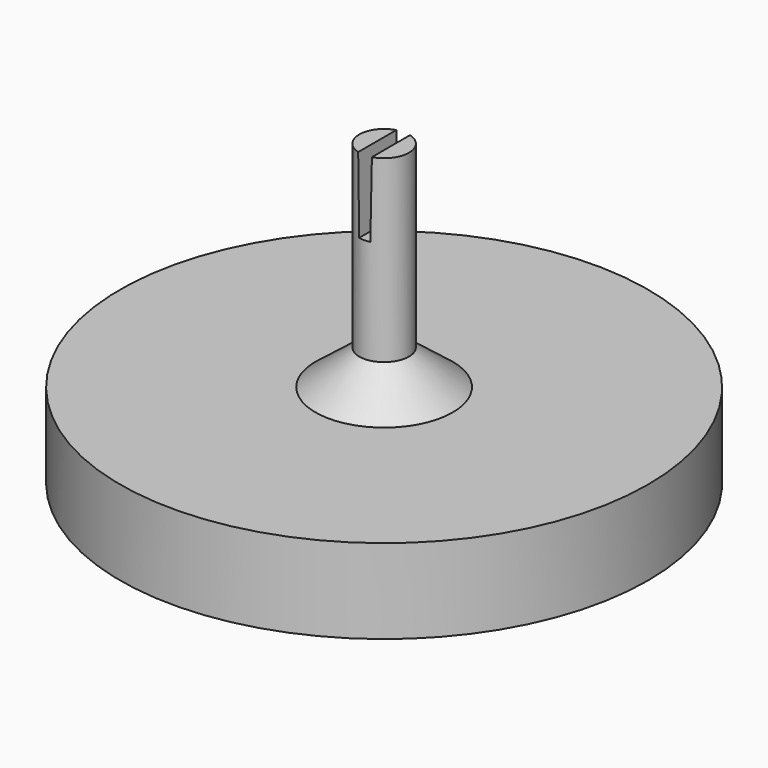
from build123d import *

# Parameters (mm, degrees)
F0_R      = 25
F1_DEPTH  = 8
F2_R      = 20.675
F3_DEPTH  = 4
F4_R      = 6.95
F5_DEPTH  = 1
F6_R      = 6.5
F7_DEPTH  = 3.3
F7_TAPER  = 52
F8_R      = 2.35
F9_DEPTH  = 17
F11_DEPTH = 7.1
F11_TAPER = 1


# Not quite as in the source:
# - a feature names something its author has since deleted; it is built from what else it names


with BuildPart() as f1:
    # F0 (on Top) → F1 (new body)
    with BuildSketch(Plane.XY):
        Circle(F0_R)
    extrude(amount=F1_DEPTH)

    # F2 (on face) → F3 (cut)
    with BuildSketch(Plane(origin=(0, 0, 0), x_dir=(1, 0, 0), z_dir=(0, 0, -1))):
        Circle(F2_R)
    extrude(amount=-F3_DEPTH, mode=Mode.SUBTRACT)

    # F4 (on face) → F5 (cut)
    with BuildSketch(Plane(origin=(0, 0, 4), x_dir=(1, 0, 0), z_dir=(0, 0, -1))):
        Circle(F4_R)
    extrude(amount=-F5_DEPTH, mode=Mode.SUBTRACT)

    # F6 (on face) → F7 (join)
    with BuildSketch(Plane.XY.offset(8)):
        Circle(F6_R)
    extrude(amount=F7_DEPTH, taper=F7_TAPER)

    # F8 (on face) → F9 (join)
    with BuildSketch(Plane.XY.offset(11.3)):
        Circle(F8_R)
    extrude(amount=F9_DEPTH)

    # F10 (on face) → F11 (cut)
    with BuildSketch(Plane.XY.offset(28.3)):
        with BuildLine():
            ThreePointArc((-0.65, 2.2583179581), (0, 2.35), (0.65, 2.2583179581))
            Line((0.65, 2.2583179581), (0.65, 4))
            Line((0.65, 4), (-0.65, 4))
            Line((-0.65, 4), (-0.65, 2.2583179581))
        make_face()
        with BuildLine():
            ThreePointArc((-0.65, -2.2583179581), (0, -2.35), (0.65, -2.2583179581))
            Line((0.65, -2.2583179581), (0.65, 2.2583179581))
            ThreePointArc((0.65, 2.2583179581), (0, 2.35), (-0.65, 2.2583179581))
            Line((-0.65, 2.2583179581), (-0.65, -2.2583179581))
        make_face()
        with BuildLine():
            Line((-0.65, -4), (0.65, -4))
            Line((0.65, -4), (0.65, -2.2583179581))
            ThreePointArc((0.65, -2.2583179581), (0, -2.35), (-0.65, -2.2583179581))
            Line((-0.65, -2.2583179581), (-0.65, -4))
        make_face()
    extrude(amount=-F11_DEPTH, taper=F11_TAPER, mode=Mode.SUBTRACT)


solid = f1.part
